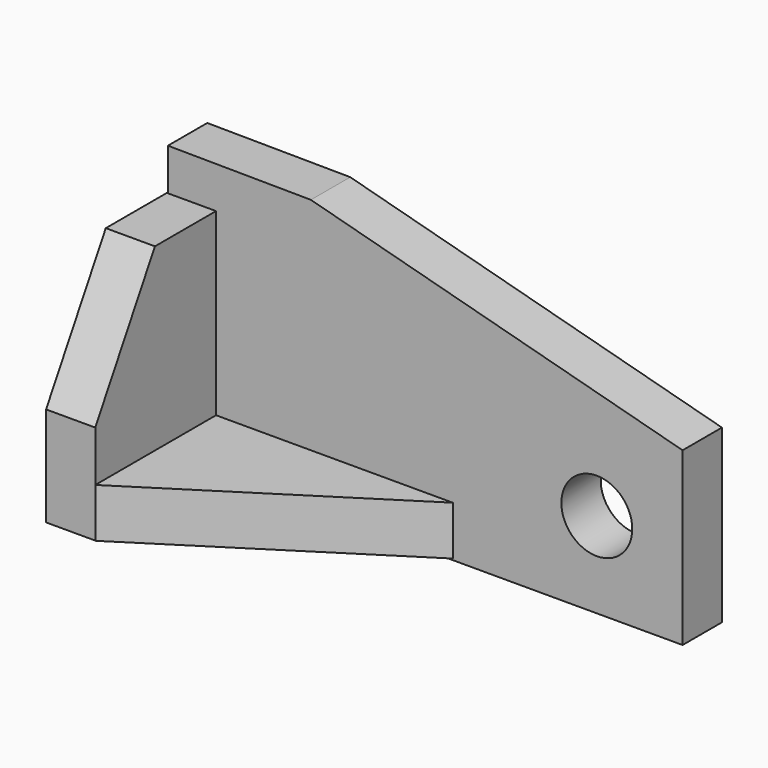
from build123d import *

# Parameters (mm, degrees)
F0_R     = 7.874
F3_DEPTH = 10.922
F4_DEPTH = 10.922
F5_DEPTH = 10.922


# Not quite as in the source:
# - a feature names something its author has since deleted; it is built from what else it names


with BuildPart() as f3:
    # F0 (on Front) → F3 (new body)
    with BuildSketch(Plane.XZ):
        Polygon((31.9869816303, 59.8861910403), (0.2369741797, 60.1518369617), (0.2369741797, -0.3118089597), (114.5369816303, -0.3118089597), (114.5369816303, 37.7669852051), align=None)
        with Locations((95.4869816303, 18.7381910403)):
            Circle(F0_R, mode=Mode.SUBTRACT)
    extrude(amount=-F3_DEPTH)

    # F1 (on Right) → F4 (join)
    with BuildSketch(Plane.YZ):
        Polygon((0, 0.0423640013), (0, 50.8423640013), (-16.9568925737, 50.8423640013), (-33.528, 22.1403640013), (-33.528, 0.0423640013), align=None)
    extrude(amount=F4_DEPTH)

    # F2 (on Top) → F5 (join)
    with BuildSketch(Plane.XY):
        Polygon((10.922, 0), (10.922, -33.528), (63.5, 0), align=None)
    extrude(amount=F5_DEPTH)


solid = f3.part
